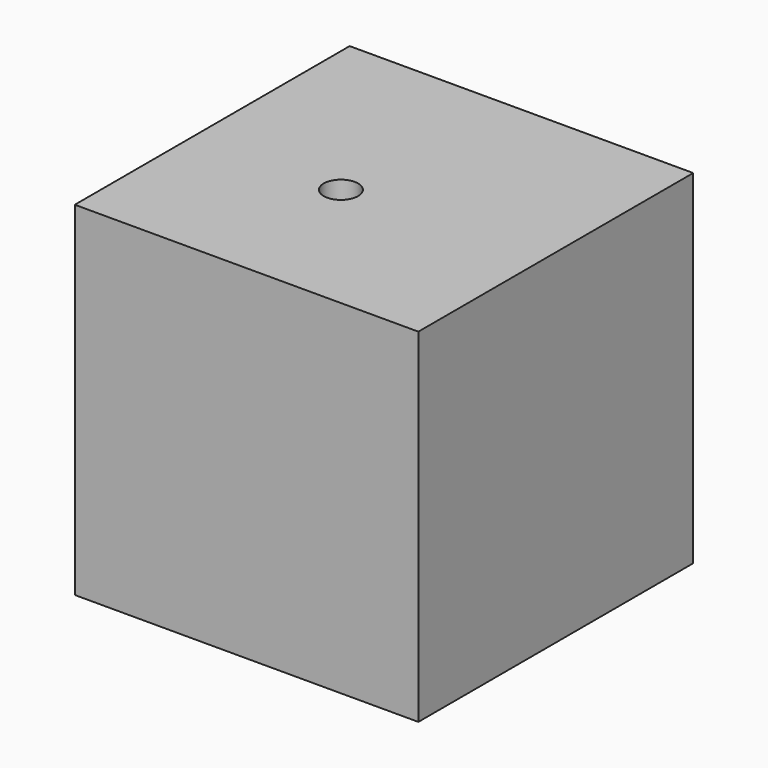
from build123d import *

# Parameters (mm, degrees)
F0_W     = 50
F0_H     = 50
F0_R     = 2.5
F1_DEPTH = 50


# Not quite as in the source:
# - a feature of the source that left no trace in its solid (it failed there, or was rolled back) is left out


with BuildPart() as f1:
    # F0 (on Top) → F1 (new body)
    with BuildSketch(Plane.XY):
        with Locations((-634.3965135887, -891.0139694249)):
            Rectangle(F0_W, F0_H)
        with Locations((-638.0807161331, -894.2453861237)):
            Circle(F0_R, mode=Mode.SUBTRACT)
    extrude(amount=F1_DEPTH)


solid = f1.part
